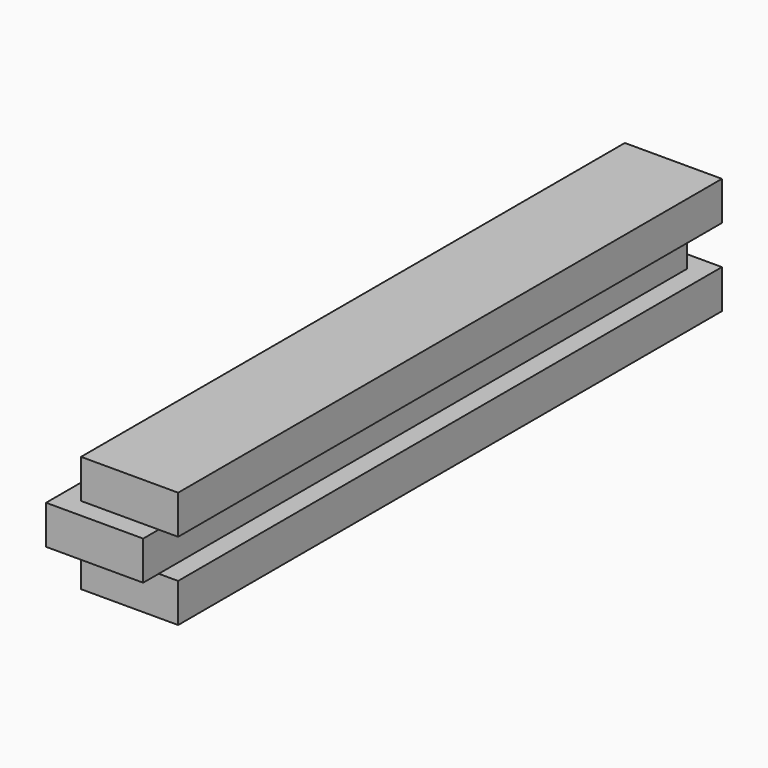
from build123d import *

# Parameters (mm, degrees)
F2_W     = 7.9375
F2_H     = 55.5625
F3_DEPTH = 3.175
F4_W     = 7.9375
F4_H     = 55.5625
F5_DEPTH = 3.175
F6_W     = 7.9375
F6_H     = 55.5625
F7_DEPTH = 3.175


# Not quite as in the source:
# - a variable given as a bare number and used for a length is read in inches; the dataset says mm whatever the document's units were


with BuildPart() as f3:
    # F2 (on Top) → F3 (new body)
    with BuildSketch(Plane.XY):
        with Locations((3.96875, 27.78125)):
            Rectangle(F2_W, F2_H)
    extrude(amount=F3_DEPTH)

    # F4 (on face) → F5 (join)
    with BuildSketch(Plane.XY.offset(3.175)):
        with Locations((2.38125, 26.19375)):
            Rectangle(F4_W, F4_H)
    extrude(amount=F5_DEPTH)

    # F6 (on face) → F7 (join)
    with BuildSketch(Plane.XY.offset(6.35)):
        with Locations((3.96875, 27.78125)):
            Rectangle(F6_W, F6_H)
    extrude(amount=F7_DEPTH)


solid = f3.part
